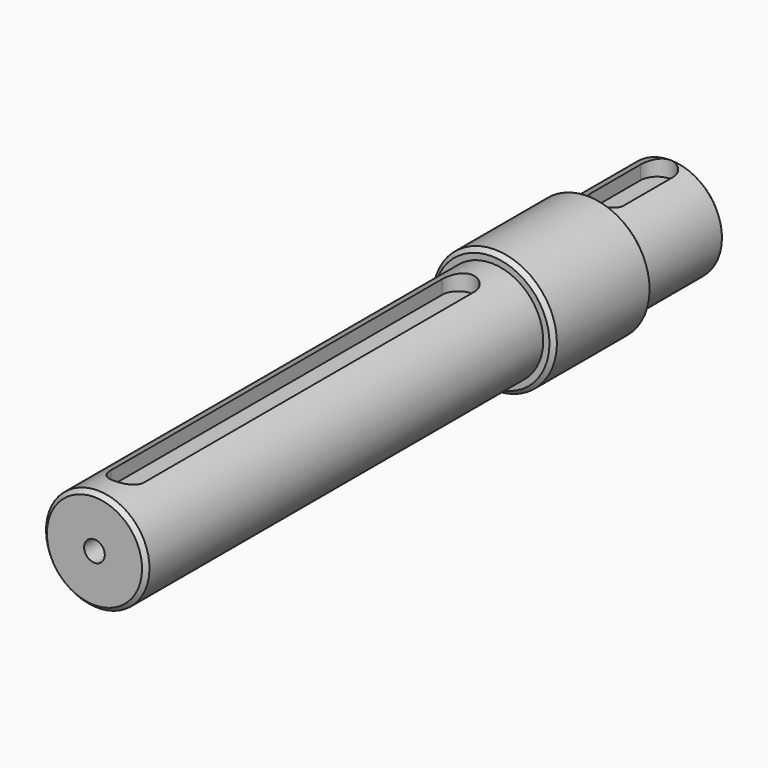
from build123d import *

# Parameters (mm, degrees)
F4_D           = 5
F4_DEPTH       = 18
F4_TIP         = 1.5021515476
F4_ON_F3_D     = 5
F4_ON_F3_DEPTH = 18
F4_ON_F3_TIP   = 1.5021515476
F5_SIZE        = 1
F8_DEPTH       = 4


with BuildPart() as f1:
    # F0 (on Right) → F1 (revolve)
    with BuildSketch(Plane.YZ):
        Polygon((-87.5, 12.5), (-87.5, 0), (87.5, 0), (87.5, 12.5), (62.5, 12.5), (62.5, 15), (32.5, 15), (32.5, 12.5), align=None)
    revolve(axis=Axis((0, 0, 0), (0, 1, 0)))

    # F4
    with Locations(Plane.XZ.offset(87.5)):
        with Locations((0, 0)):
            Hole(F4_D / 2, depth=F4_DEPTH)
            with Locations((0, 0, -(F4_DEPTH + F4_TIP / 2))):  # 118° drill point
                Cone(0, F4_D / 2, F4_TIP, mode=Mode.SUBTRACT)

    # F4 on F3
    with Locations(Plane(origin=(0, 87.5, 0), x_dir=(-1, 0, 0), z_dir=(0, 1, 0))):
        with Locations((0, 0)):
            Hole(F4_ON_F3_D / 2, depth=F4_ON_F3_DEPTH)
            with Locations((0, 0, -(F4_ON_F3_DEPTH + F4_ON_F3_TIP / 2))):  # 118° drill point
                Cone(0, F4_ON_F3_D / 2, F4_ON_F3_TIP, mode=Mode.SUBTRACT)

    # F5
    f5_edges = [f1.edges().sort_by_distance(p)[0] for p in [
        (0, -87.5, -12.5),
        (0, 87.5, -12.5),
        (0, 32.5, -15),
        (0, 62.5, -15),
    ]]
    chamfer(f5_edges, length=F5_SIZE)

    # F7 (on offset) → F8 (cut)
    with BuildSketch(Plane.XY.offset(12.5)):
        with BuildLine():
            ThreePointArc((-4, -77.5), (0, -81.5), (4, -77.5))
            Line((4, -77.5), (4, 22.5))
            ThreePointArc((4, 22.5), (0, 26.5), (-4, 22.5))
            Line((-4, 22.5), (-4, -77.5))
        make_face()
        with BuildLine():
            ThreePointArc((-4, 67.5), (0, 63.5), (4, 67.5))
            Line((4, 67.5), (4, 82.5))
            ThreePointArc((4, 82.5), (0, 86.5), (-4, 82.5))
            Line((-4, 82.5), (-4, 67.5))
        make_face()
    extrude(amount=-F8_DEPTH, mode=Mode.SUBTRACT)


solid = f1.part
